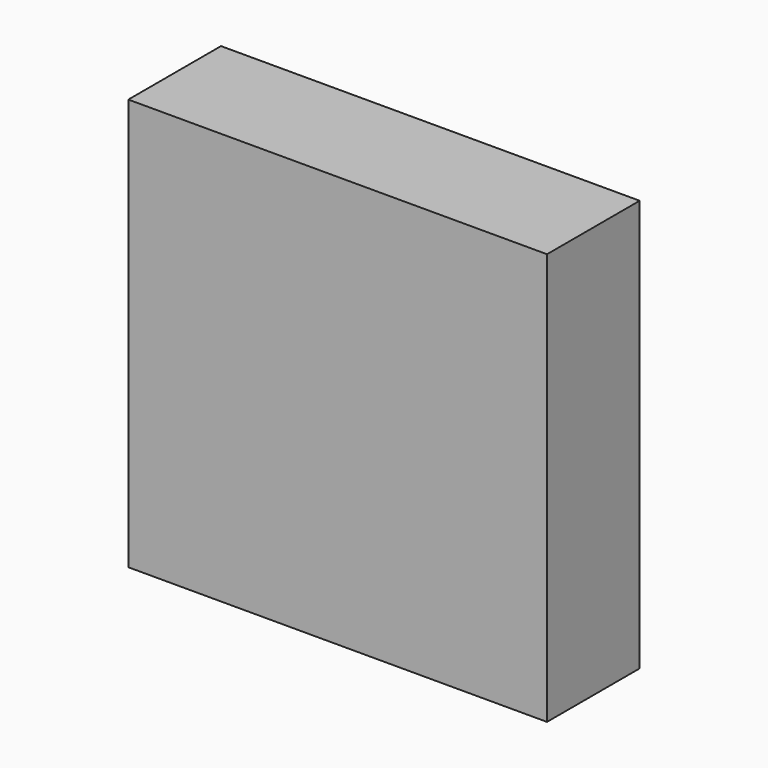
from build123d import *

# Parameters (mm, degrees)
F0_W     = 27.7622193098
F0_H     = 27.1012242883
F1_DEPTH = 5
F3_T     = 6


# Not quite as in the source:
# - a feature of the source that left no trace in its solid (it failed there, or was rolled back) is left out


with BuildPart() as f1:
    # F0 (on Front) → F1 (new body)
    with BuildSketch(Plane.XZ):
        Rectangle(F0_W, F0_H)
    extrude(amount=F1_DEPTH)

    # F3
    f3_openings = [f1.faces().sort_by_distance(p)[0] for p in [
        (0, 0, 0),
    ]]
    offset(amount=F3_T, openings=f3_openings, kind=Kind.INTERSECTION)


solid = f1.part
